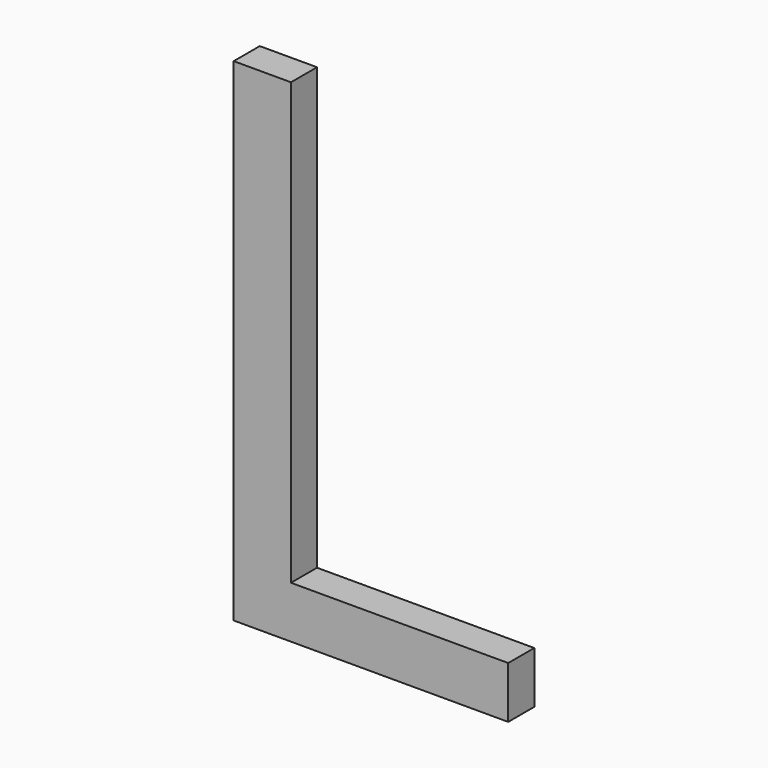
from build123d import *

# Parameters (mm, degrees)
F0_TEXT_SIZE = 53.7637155503
F1_DEPTH     = 2.54


# Not quite as in the source:
# - Text() gives the source's letters only with a copy of the font that has no kerning and outlines rounded to 1/6400 em; it was checked with that copy


with BuildPart() as f1:
    # F0 (on Front) → F1 (new body)
    with BuildSketch(Plane.XZ):
        with Locations((-38.1342619658, 0)):
            Text('L', F0_TEXT_SIZE, font='Open Sans', text_align=(TextAlign.LEFT, TextAlign.BOTTOM))
    extrude(amount=F1_DEPTH)


solid = f1.part
